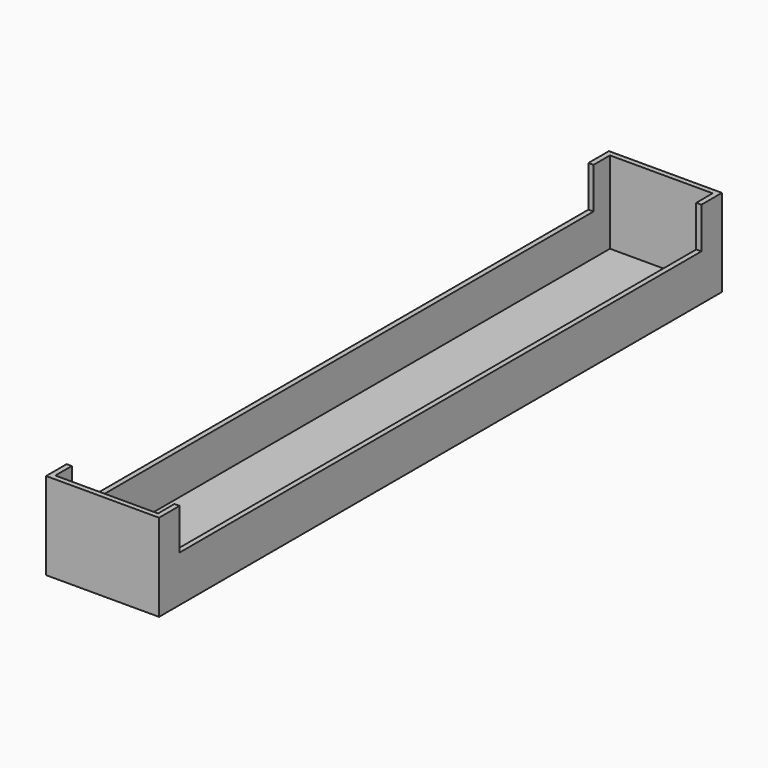
from build123d import *

# Parameters (mm, degrees)
F0_W         = 22
F0_H         = 137
F1_DEPTH     = 1
F2_W         = 1
F2_H         = 4
F3_DEPTH     = 16
F4_W         = 1
F4_H         = 127
F5_DEPTH     = 8
F6_TEXT_SIZE = 13.8888888889
F7_DEPTH     = 0.5


# Not quite as in the source:
# - Text() gives the source's letters only with a copy of the font that has no kerning and outlines rounded to 1/6400 em; it was checked with that copy


with BuildPart() as f1:
    # F0 (on Top) → F1 (new body)
    with BuildSketch(Plane.XY):
        Rectangle(F0_W, F0_H)
    extrude(amount=F1_DEPTH)

    # F2 (on face) → F3 (join)
    with BuildSketch(Plane.XY.offset(1)):
        Polygon((11, 68.5), (-11, 68.5), (-11, 67.5), (-10, 67.5), (10, 67.5), (11, 67.5), align=None)
        with Locations((-10.5, 65.5)):
            Rectangle(F2_W, F2_H)
        with Locations((10.5, 65.5)):
            Rectangle(F2_W, F2_H)
        Polygon((-11, -67.5), (-11, -68.5), (11, -68.5), (11, -67.5), (10, -67.5), (-10, -67.5), align=None)
        with Locations((-10.5, -65.5)):
            Rectangle(F2_W, F2_H)
        with Locations((10.5, -65.5)):
            Rectangle(F2_W, F2_H)
    extrude(amount=F3_DEPTH)

    # F4 (on face) → F5 (join)
    with BuildSketch(Plane.XY.offset(1)):
        with Locations((10.5, 0)):
            Rectangle(F4_W, F4_H)
        with Locations((-10.5, 0)):
            Rectangle(F4_W, F4_H)
    extrude(amount=F5_DEPTH)

    # F6 (on face) → F7 (cut)
    with BuildSketch(Plane(origin=(0, 0, 0), x_dir=(1, 0, 0), z_dir=(0, 0, -1))):
        with Locations(Location((-5, 64.5), (0, 0, -90))):
            Text('Guard', F6_TEXT_SIZE, font='Open Sans', font_style=FontStyle.BOLD, text_align=(TextAlign.LEFT, TextAlign.BOTTOM))
    extrude(amount=-F7_DEPTH, mode=Mode.SUBTRACT)


solid = f1.part
